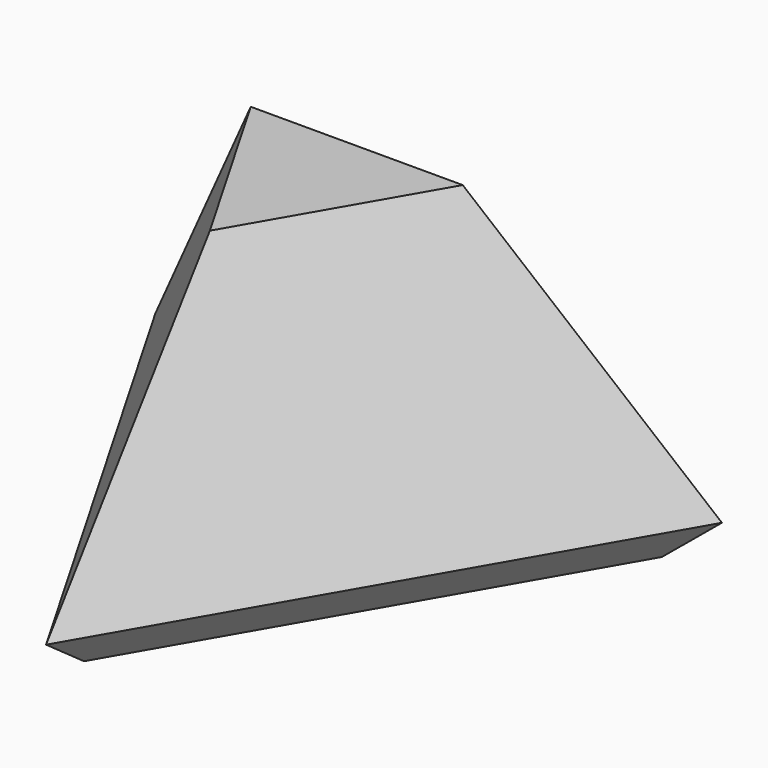
from build123d import *

# Parameters (mm, degrees)
F1_DEPTH = 87.5
F1_TAPER = 20
F2_SIZE  = 10


with BuildPart() as f1:
    # F0 (on Top) → F1 (new body)
    with BuildSketch(Plane.XY):
        Polygon((84.5943443278, 48.8405674696), (-84.5943443278, 48.8405674696), (0, -97.6811349392), align=None)
    extrude(amount=F1_DEPTH, taper=F1_TAPER)

    # F2
    f2_edges = [f1.edges().sort_by_distance(p)[0] for p in [
        (42.297172, -24.420284, 0),
        (-42.297172, -24.420284, 0),
        (0, 48.840567, 0),
    ]]
    chamfer(f2_edges, length=F2_SIZE)


solid = f1.part
